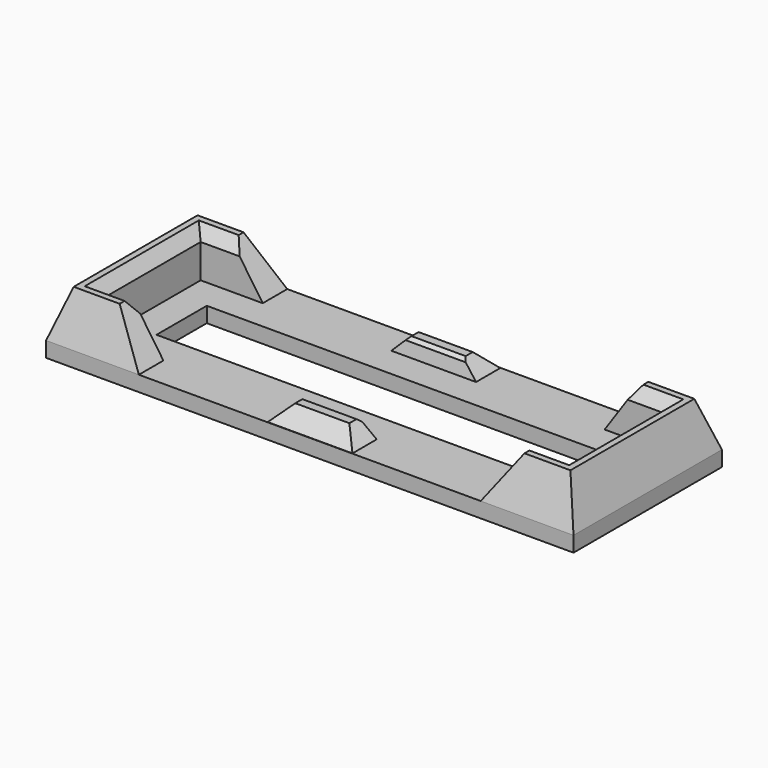
from build123d import *

# Parameters (mm, degrees)
F0_W      = 172
F0_H      = 60.5
F4_DEPTH  = 5
F6_SIZE2  = 4
F6_SIZE   = 3
F9_DEPTH  = 5
F10_SIZE  = 4.99999
F11_SIZE2 = 0.99999
F11_SIZE  = 4.99999
F12_SIZE  = 1
F14_W     = 132
F14_H     = 20.5
F15_DEPTH = 12.5


# Not quite as in the source:
# - a fillet or chamfer is up to 0.001 mm smaller than in the source, because OpenCascade refuses the exact size


with BuildPart() as f4:
    # F0 (on Top) → F4 (new body)
    with BuildSketch(Plane.XY):
        Rectangle(F0_W, F0_H)
    extrude(amount=-F4_DEPTH)

    # F3 (on Top) → F5 section 0
    with BuildSketch(Plane.XY):
        Polygon((-86, 0), (-86, -30.25), (-55.75, -30.25), (-55.75, -20.25), (-76, -20.25), (-76, 0), align=None)
    # F2 (on offset) → F5 section 1
    with BuildSketch(Plane.XY.offset(15)):
        Polygon((-76, -20.25), (-76, 0), (-81, 0), (-81, -25.25), (-66, -25.25), (-66, -20.25), align=None)
    loft()

    # F6
    f6_edges = [f4.edges().sort_by_distance(p)[0] for p in [
        (-76, -10.125, 15),
        (-71, -20.25, 15),
    ]]
    chamfer(f6_edges, length=F6_SIZE, length2=F6_SIZE2)

    # F7: F4 across plane


with BuildPart() as f4_1:
    add(f4.part)
    add(f4.part.mirror(Plane.YZ))

    # F8 (on face) → F9 (join)
    with BuildSketch(Plane.XY):
        Polygon((13.8189587742, -20.25), (0, -20.25), (-13.8189587742, -20.25), (-13.8189587742, -30.1344580948), (0, -30.1344580948), (13.8189587742, -30.1344580948), align=None)
    extrude(amount=F9_DEPTH)

    # F10 (size 5 in the source; OpenCascade refuses exactly that, so slightly less here)
    f10_edges = [f4_1.edges().sort_by_distance(p)[0] for p in [
        (13.818959, -25.192229, 5),
        (0, -30.134458, 5),
        (-13.818959, -25.192229, 5),
    ]]
    chamfer(f10_edges, length=F10_SIZE)

    # F11 (size 5 and 1 in the source; OpenCascade refuses exactly that, so slightly less here)
    f11_edges = [f4_1.edges().sort_by_distance(p)[0] for p in [
        (0, -20.25, 5),
    ]]
    f11_side = f4_1.faces().sort_by_distance((0, -20.25, 2.315943))[0]
    chamfer(f11_edges, length=F11_SIZE, length2=F11_SIZE2, reference=f11_side)

    # F12
    f12_edges = [f4_1.edges().sort_by_distance(p)[0] for p in [
        (0, -21.24999, 5),
    ]]
    chamfer(f12_edges, length=F12_SIZE)

    # F13: F4 across plane


with BuildPart() as f4_2:
    add(f4_1.part)
    add(f4_1.part.mirror(Plane.XZ))

    # F14 (on Top) → F15 (cut, symmetric)
    with BuildSketch(Plane.XY):
        Rectangle(F14_W, F14_H)
    extrude(amount=F15_DEPTH, both=True, mode=Mode.SUBTRACT)


solid = f4_2.part
